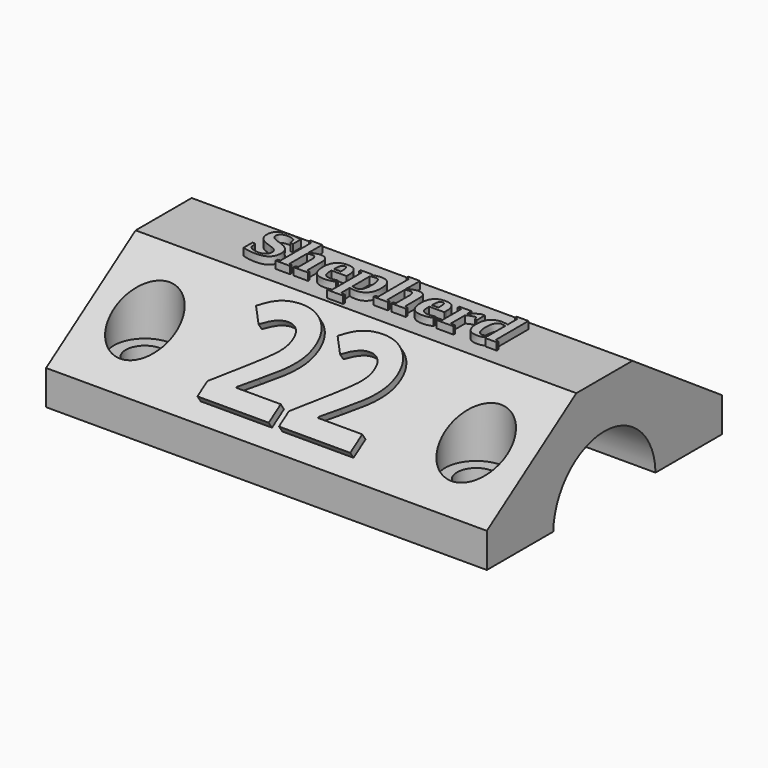
from build123d import *

# Parameters (mm, degrees)
F0_W           = 76.2
F0_H           = 19.05
F1_DEPTH       = 25.4
F3_DEPTH       = 76.2
F4_START       = -25.4
F4_DEPTH       = 25.4
F6_D           = 6.604
F6_CBORE_D     = 10.7442
F6_CBORE_DEPTH = 12.192
F8_DEPTH       = 76.2
F9_TEXT_SIZE   = 10.8607114624
F10_DEPTH      = 1.27
F11_TEXT_SIZE  = 24.6944444444
F12_DEPTH      = 1.27


# Not quite as in the source:
# - a feature names something its author has since deleted; it is built from what else it names
# - Text() gives the source's letters only with a copy of the font that has no kerning and outlines rounded to 1/6400 em; it was checked with that copy


with BuildPart() as f1:
    # F0 (on Front) → F1 (new body, symmetric)
    with BuildSketch(Plane.XZ):
        Rectangle(F0_W, F0_H)
    extrude(amount=F1_DEPTH, both=True)

    # F2 (on face) → F3 (cut)
    with BuildSketch(Plane.YZ.offset(38.1)):
        with BuildLine():
            Line((-11.049, -9.525), (11.049, -9.525))
            ThreePointArc((11.049, -9.525), (7.7235423544, -1.8767154726), (0, 1.27))
            ThreePointArc((0, 1.27), (-7.7235423544, -1.8767154726), (-11.049, -9.525))
        make_face()
    extrude(amount=-F3_DEPTH, mode=Mode.SUBTRACT)

    # F2 (on face) → F4 (cut)
    with BuildSketch(Plane.YZ.offset(38.1).offset(F4_START)):
        with BuildLine():
            Line((-12.1256774291, -9.525), (-11.049, -9.525))
            ThreePointArc((-11.049, -9.525), (-7.7235423544, -1.8767154726), (0, 1.27))
            Line((0, 1.27), (0, 2.3389752023))
            ThreePointArc((0, 2.3389752023), (-8.4853122439, -1.1171025881), (-12.1256774291, -9.525))
        make_face()
        with BuildLine():
            ThreePointArc((0, 1.27), (7.7235423544, -1.8767154726), (11.049, -9.525))
            Line((11.049, -9.525), (12.1033722535, -9.525))
            ThreePointArc((12.1033722535, -9.525), (8.4709751039, -1.1249058342), (0, 2.3389752023))
            Line((0, 2.3389752023), (0, 1.27))
        make_face()
        with BuildLine():
            Line((-11.049, -9.525), (11.049, -9.525))
            ThreePointArc((11.049, -9.525), (7.7235423544, -1.8767154726), (0, 1.27))
            ThreePointArc((0, 1.27), (-7.7235423544, -1.8767154726), (-11.049, -9.525))
        make_face()
    extrude(amount=-F4_DEPTH, mode=Mode.SUBTRACT)

    # F6 (through all)
    with Locations(Plane.XY.offset(9.525)):
        with Locations((-28.6385, 15.875), (-28.6385, -15.875), (28.6385, -15.875), (28.6385, 15.875)):
            CounterBoreHole(F6_D / 2, F6_CBORE_D / 2, F6_CBORE_DEPTH)

    # F7 (on face) → F8 (cut)
    with BuildSketch(Plane(origin=(-38.1, 0, 0), x_dir=(0, -1, 0), z_dir=(-1, 0, 0))):
        Polygon((-25.4, 9.525), (-25.4, -3.5569551401), (-6.0592088848, 9.525), align=None)
        Polygon((25.4, 9.525), (6.0592088848, 9.525), (25.4, -3.5569551401), align=None)
    extrude(amount=-F8_DEPTH, mode=Mode.SUBTRACT)

    # F9 (on face) → F10 (join)
    with BuildSketch(Plane.XY.offset(9.525)):
        with Locations((-22.606, -3.0577247253)):
            Text('Shepherd', F9_TEXT_SIZE, font='Tinos', font_style=FontStyle.BOLD, text_align=(TextAlign.LEFT, TextAlign.BOTTOM))
    extrude(amount=F10_DEPTH)

    # F11 (on face) → F12 (join)
    with BuildSketch(Plane(origin=(0, -6.3222776401, 9.3470624154), x_dir=(1, 0, 0), z_dir=(0, -0.5602646712, 0.8283136472))):
        with Locations((-14.5041276042, -19.7868698242)):
            Text('22', F11_TEXT_SIZE, font='Open Sans', font_style=FontStyle.BOLD, text_align=(TextAlign.LEFT, TextAlign.BOTTOM))
    extrude(amount=F12_DEPTH)


solid = f1.part
